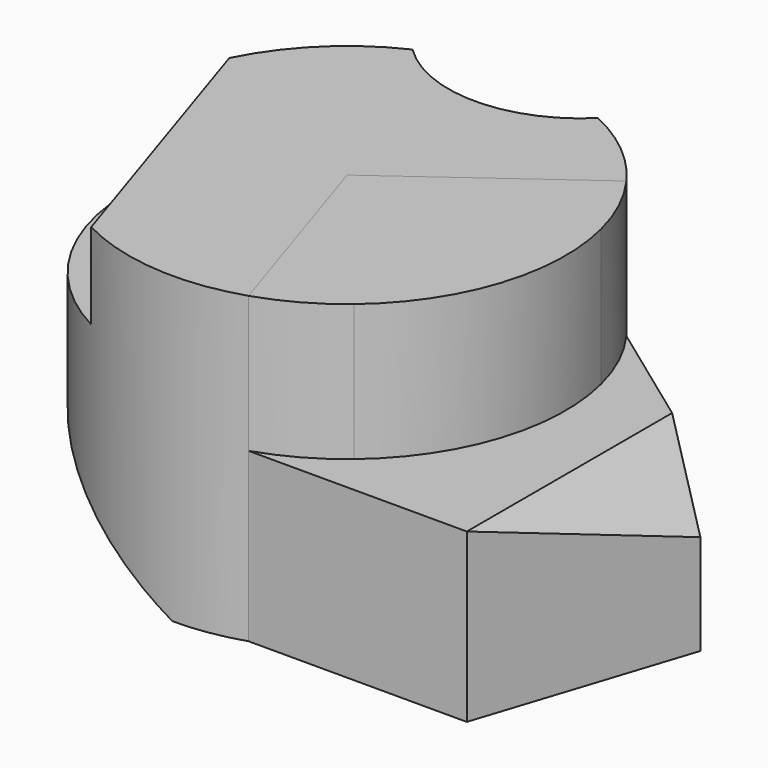
from build123d import *

# Parameters (mm, degrees)
F1_DEPTH  = 78
F2_DEPTH  = 43
F4_DEPTH  = 22
F7_DEPTH  = 56
F11_DEPTH = 15
F12_DEPTH = 78
F13_DEPTH = 21
F14_DEPTH = 15


with BuildPart() as f1:
    # F0 (on Top) → F1 (new body)
    with BuildSketch(Plane.XY):
        with BuildLine():
            Line((17.304951685, -53.2591649125), (0, 0))
            Line((0, 0), (45.304951685, 32.9159741284))
            ThreePointArc((45.304951685, 32.9159741284), (35.6688410129, 43.1709830882), (23.7804541588, 50.7))
            ThreePointArc((23.7804541588, 50.7), (0, 41), (-23.7804541588, 50.7))
            ThreePointArc((-23.7804541588, 50.7), (-52.0803228235, -20.5825162359), (17.304951685, -53.2591649125))
        make_face()
    extrude(amount=F1_DEPTH)

    # F3 (on face) → F4 (cut)
    with BuildSketch(Plane.XY.offset(78)):
        with BuildLine():
            ThreePointArc((-50.1532039809, 24.9129711286), (-53.2591649125, -17.304951685), (-25.9313173227, -49.6343306786))
            Line((-25.9313173227, -49.6343306786), (-50.1532039809, 24.9129711286))
        make_face()
    extrude(amount=-F4_DEPTH, mode=Mode.SUBTRACT)

    # F6 (on offset) → F7 (cut)
    with BuildSketch(Plane.XZ.offset(56)):
        Polygon((-56, 0), (0, 0), (-56, 32.3316150746), align=None)
    extrude(amount=-F7_DEPTH, mode=Mode.SUBTRACT)

    # F10 (on face) → F14 (cut)
    with BuildSketch(Plane(origin=(58.1524758425, 0, 58.1524758425), x_dir=(0.7071067812, 0, -0.7071067812), z_dir=(-0.7071067812, 0, -0.7071067812))):
        Polygon((21.42883684, -12.5727833442), (45.9017342091, 0), (21.42883684, 53.2591649125), align=None)
    extrude(amount=-F14_DEPTH, mode=Mode.SUBTRACT)


with BuildPart() as f1b:
    # F0 (on Top) → F1, piece 2 (new body)
    with BuildSketch(Plane.XY):
        with BuildLine():
            ThreePointArc((36.0143064054, -42.8832103992), (53.2591649125, -17.304951685), (54.3423045662, 13.5245678096))
            Line((54.3423045662, 13.5245678096), (24.6869805963, -8.0212862363))
            Line((24.6869805963, -8.0212862363), (36.0143064054, -42.8832103992))
        make_face()
    extrude(amount=F1_DEPTH)

    # F0 (on Top) → F2 (join)
    with BuildSketch(Plane.XY):
        with BuildLine():
            Line((90.60990337, 0), (45.304951685, 32.9159741284))
            ThreePointArc((45.304951685, 32.9159741284), (50.7582562678, 23.6558538347), (54.3423045662, 13.5245678096))
            ThreePointArc((54.3423045662, 13.5245678096), (53.2591649125, -17.304951685), (36.0143064054, -42.8832103992))
            ThreePointArc((36.0143064054, -42.8832103992), (27.1597299111, -48.972942235), (17.304951685, -53.2591649125))
            Line((17.304951685, -53.2591649125), (73.304951685, -53.2591649125))
            Line((73.304951685, -53.2591649125), (90.60990337, 0))
        make_face()
    extrude(amount=F2_DEPTH)

    # F10 (on face) → F11 (cut)
    with BuildSketch(Plane(origin=(58.1524758425, 0, 58.1524758425), x_dir=(0.7071067812, 0, -0.7071067812), z_dir=(-0.7071067812, 0, -0.7071067812))):
        Polygon((21.42883684, -12.5727833442), (45.9017342091, 0), (21.42883684, 53.2591649125), align=None)
    extrude(amount=-F11_DEPTH, mode=Mode.SUBTRACT)

    # F0 (on Top) → F12 (join)
    with BuildSketch(Plane.XY):
        with BuildLine():
            Line((45.304951685, 32.9159741284), (0, 0))
            Line((0, 0), (17.304951685, -53.2591649125))
            ThreePointArc((17.304951685, -53.2591649125), (27.1597299111, -48.972942235), (36.0143064054, -42.8832103992))
            Line((36.0143064054, -42.8832103992), (24.6869805963, -8.0212862363))
            Line((24.6869805963, -8.0212862363), (54.3423045662, 13.5245678096))
            ThreePointArc((54.3423045662, 13.5245678096), (50.7582562678, 23.6558538347), (45.304951685, 32.9159741284))
        make_face()
    extrude(amount=F12_DEPTH)

    # F0 (on Top) → F13 (cut)
    with BuildSketch(Plane.XY):
        with BuildLine():
            Line((45.304951685, 32.9159741284), (0, 0))
            Line((0, 0), (17.304951685, -53.2591649125))
            ThreePointArc((17.304951685, -53.2591649125), (27.1597299111, -48.972942235), (36.0143064054, -42.8832103992))
            Line((36.0143064054, -42.8832103992), (24.6869805963, -8.0212862363))
            Line((24.6869805963, -8.0212862363), (54.3423045662, 13.5245678096))
            ThreePointArc((54.3423045662, 13.5245678096), (50.7582562678, 23.6558538347), (45.304951685, 32.9159741284))
        make_face()
    extrude(amount=F13_DEPTH, mode=Mode.SUBTRACT)


solid = Compound([f1.part, f1b.part])
